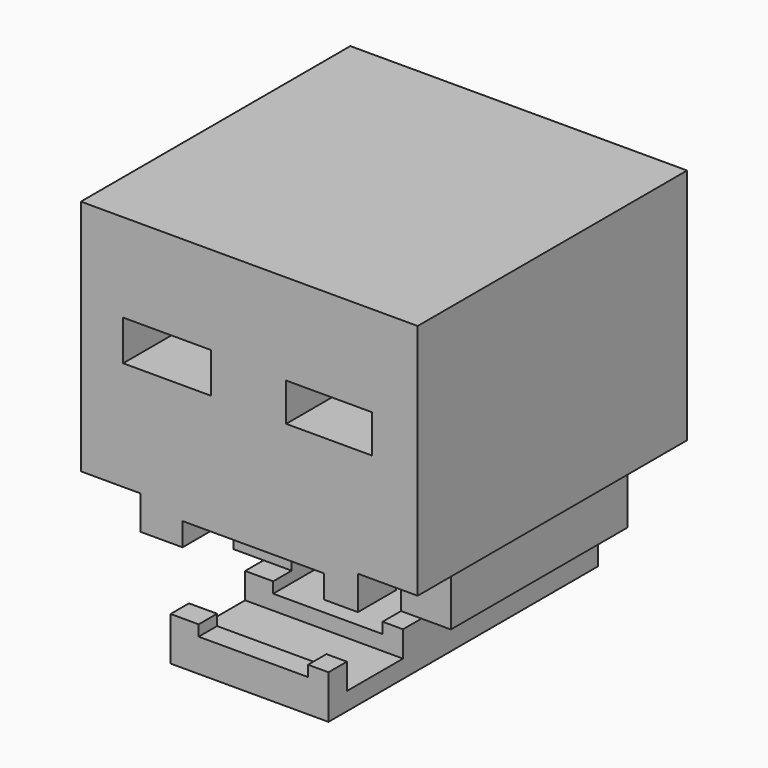
from build123d import *

# Parameters (mm, degrees)
F1_DEPTH  = 29.21
F2_W      = 15.2287210607
F2_H      = 6.9798285036
F2_W_2    = 14.8809022204
F2_H_2    = 6.6161153238
F3_DEPTH  = 12.7
F5_DEPTH  = 58.42
F7_DEPTH  = 37.677641958
F8_W      = 12.1679750076
F8_H      = 4.4820662588
F9_DEPTH  = 27.3915433795
F11_DEPTH = 14.224
F13_DEPTH = 14.224


# Not quite as in the source:
# - a feature names something its author has since deleted; it is built from what else it names


with BuildPart() as f1:
    # F0 (on Front) → F1 (new body, symmetric)
    with BuildSketch(Plane.XZ):
        Polygon((29.21, 29.21), (-29.21, 29.21), (-29.21, -11.9885886088), (-18.838820979, -11.9885886088), (-18.838820979, -28.7043564022), (-13.6548336595, -28.7043564022), (-13.6548336595, -36.2838581204), (13.73670972, -36.2838581204), (13.73670972, -28.7043564022), (18.838820979, -28.7043564022), (18.838820979, -11.9885886088), (29.21, -11.9885886088), align=None)
    extrude(amount=F1_DEPTH, both=True)

    # F2 (on face) → F3 (cut)
    with BuildSketch(Plane.XZ.offset(29.21)):
        with Locations((-14.2686051116, 10.3913402672)):
            Rectangle(F2_W, F2_H)
        with Locations((13.8336278745, 10.1568780676)):
            Rectangle(F2_W_2, F2_H_2)
    extrude(amount=-F3_DEPTH, mode=Mode.SUBTRACT)

    # F4 (on face) → F5 (cut, through all)
    with BuildSketch(Plane.XZ.offset(29.21)):
        Polygon((-11.5834288299, -13.842545168), (-11.5834288299, -24.4784541428), (-8.7825786322, -24.4784541428), (-8.7825786322, -30.5909998715), (10.1944149937, -30.5909998715), (10.1944149937, -24.4784541428), (12.9711292684, -24.4784541428), (12.9711292684, -13.8473447557), align=None)
    extrude(amount=-F5_DEPTH, mode=Mode.SUBTRACT)

    # F6 (on face) → F7 (cut, through all)
    with BuildSketch(Plane(origin=(-18.838820979, 0, 0), x_dir=(0, -1, 0), z_dir=(-1, 0, 0))):
        Polygon((20.9785699844, -12.4480193481), (-1.9933339208, -12.4480193481), (-1.9933339208, -17.8599096835), (9.0442672372, -17.8599096835), (9.0442672372, -28.7043564022), (29.3133463711, -28.7043564022), (29.3133463711, -17.8599096835), (20.9785699844, -17.8599096835), align=None)
    extrude(amount=-F7_DEPTH, mode=Mode.SUBTRACT)

    # F8 (on face) → F9 (cut, through all)
    with BuildSketch(Plane.YZ.offset(13.73670972)):
        with Locations((-19.1350400816, -30.9453895316)):
            Rectangle(F8_W, F8_H)
    extrude(amount=-F9_DEPTH, mode=Mode.SUBTRACT)

    # F10 (on face) → F11 (join)
    with BuildSketch(Plane(origin=(0, 29.21, 0), x_dir=(-1, 0, 0), z_dir=(0, 1, 0))):
        Polygon((12.8193823621, -11.6105714807), (-15.3379710391, -11.6105714807), (-15.3379710391, -26.3032335788), (-12.9711292684, -26.3032335788), (-12.9795083776, -31.884662807), (10.1667114277, -31.884662807), (10.1667114277, -26.3032335788), (12.8193823621, -26.3032335788), align=None)
    extrude(amount=-F11_DEPTH)

    # F12 (on face) → F13 (cut, through all)
    with BuildSketch(Plane(origin=(0, 29.21, 0), x_dir=(-1, 0, 0), z_dir=(0, 1, 0))):
        Polygon((6.527592428, -23.4476383775), (6.527592428, -16.5502689779), (-8.1549943425, -16.5502689779), (-8.1549943425, -23.4476383775), (-5.1418524235, -23.4476383775), (-5.1418524235, -28.0656591058), (3.516294295, -28.0656591058), (3.516294295, -23.4476383775), align=None)
    extrude(amount=-F13_DEPTH, mode=Mode.SUBTRACT)


solid = f1.part
